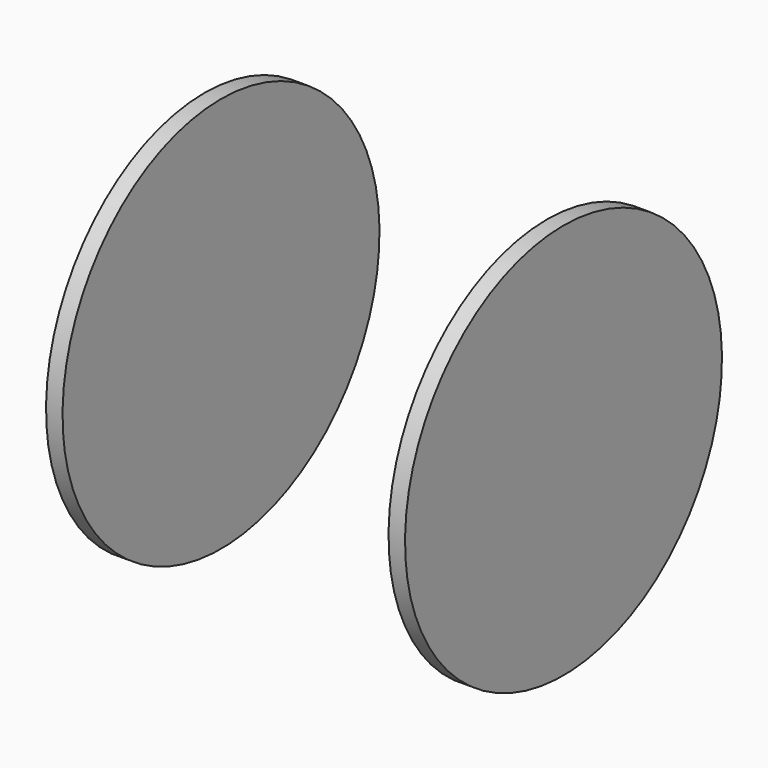
from build123d import *


# Not quite as in the source:
# - a feature of the source that left no trace in its solid (it failed there, or was rolled back) is left out
# - the program builds the solid bodies; features that only make, move or delete a surface that nothing else refers to are left out


with BuildPart() as f2:
    # F0 (on Front) → F2 (revolve)
    with BuildSketch(Plane.XZ):
        Polygon((-34.5258565417, 0), (-31.3508565417, 0), (-31.3508565417, 25.4), (-31.3508565417, 38.1), (-34.5258565417, 38.1), align=None)
    revolve(axis=Axis((0.2852417529, 0, 0), (1, 0, 0)))


with BuildPart() as f2b:
    # F0 (on Front) → F2, piece 2 (revolve)
    with BuildSketch(Plane.XZ):
        Polygon((31.3508565417, 25.4), (31.3508565417, 0), (34.5258565417, 0), (34.5258565417, 38.1), (31.3508565417, 38.1), align=None)
    revolve(axis=Axis((0.2852417529, 0, 0), (1, 0, 0)))


solid = Compound([f2.part, f2b.part])
